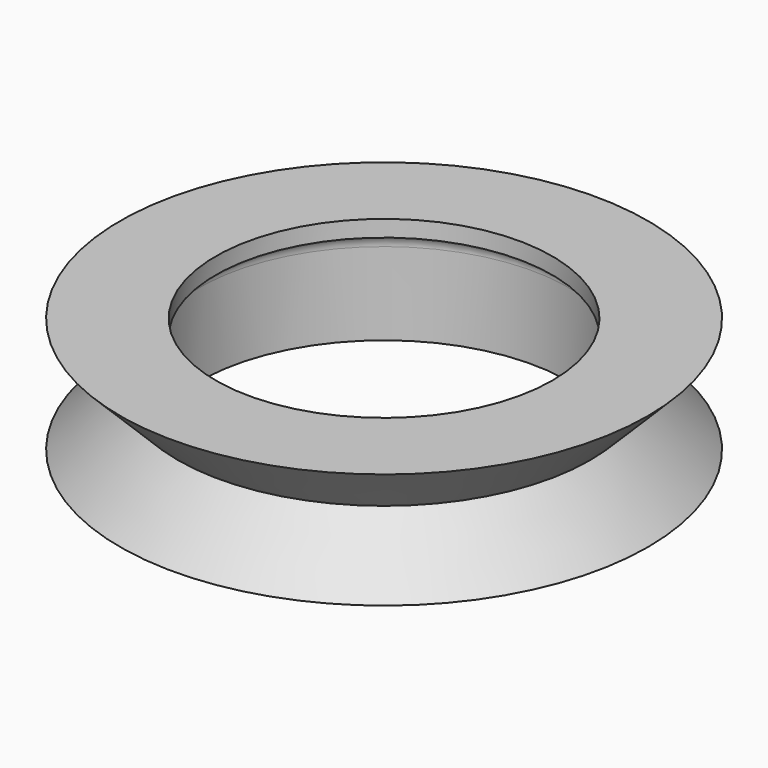
from build123d import *

# Parameters (mm, degrees)
F0_W = 1
F0_H = 1
F3_R = 0.99999


# Not quite as in the source:
# - a fillet or chamfer is up to 0.001 mm smaller than in the source, because OpenCascade refuses the exact size


with BuildPart() as f1:
    # F0 (on Front) → F1 (revolve)
    with BuildSketch(Plane.XZ):
        Polygon((16, 3.5), (11.2, 3.5), (11.2, 2.5), (11.2, -3.5), (16, -3.5), (12.5, 0), align=None)
        Polygon((10.2, 3.5), (0, 3.5), (0, -3.5), (11.2, -3.5), (11.2, 2.5), (10.2, 2.5), align=None)
        with Locations((10.7, 3)):
            Rectangle(F0_W, F0_H)
    revolve(axis=Axis((0, 0, -0.2485097927), (0, 0, -1)))

    # F0 (on Front) → F2 (revolve, cut)
    with BuildSketch(Plane.XZ):
        Polygon((10.2, 3.5), (0, 3.5), (0, -3.5), (11.2, -3.5), (11.2, 2.5), (10.2, 2.5), align=None)
    revolve(axis=Axis((0, 0, -0.2485097927), (0, 0, -1)), mode=Mode.SUBTRACT)

    # F3 (radius 1 in the source; OpenCascade refuses exactly that, so slightly less here)
    f3_edges = [f1.edges().sort_by_distance(p)[0] for p in [
        (-11.2, 0, 2.5),
    ]]
    fillet(f3_edges, radius=F3_R)


solid = f1.part
